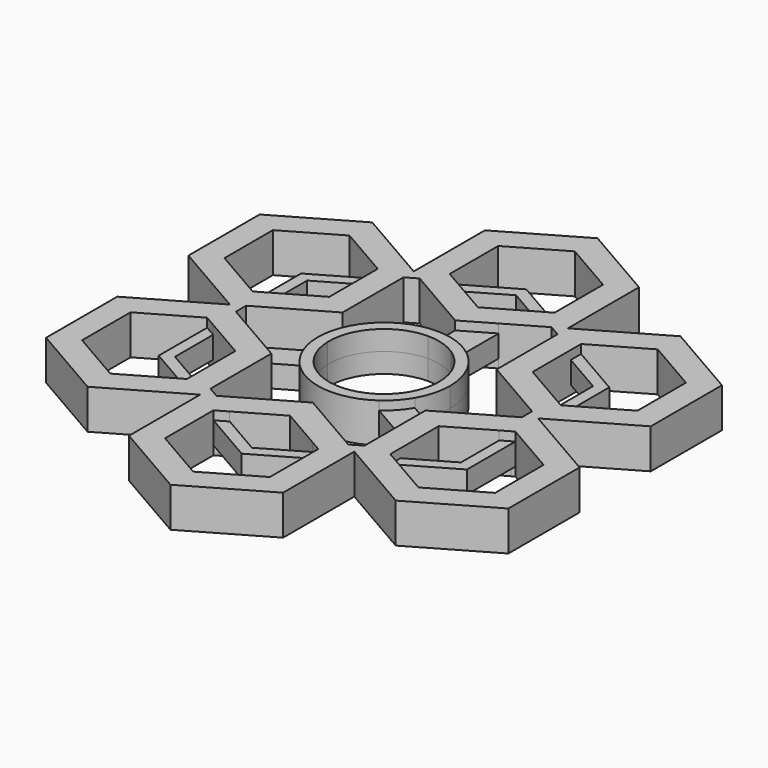
from build123d import *
from build123d import SkipClean  # not in build123d's __all__

# Parameters (mm, degrees)
F1_DEPTH      = 4.572
F1_DEPTH_BACK = 4.572
F4_DEPTH      = 2.032
F6_DEPTH      = 2.032


# Not quite as in the source:
# - after a boolean that leaves OpenCascade's solid faulty, fix() repairs it


with BuildPart() as f1:
    # F0 (on Top) → F1 (new body, two sides)
    with BuildSketch(Plane.XY) as f1_sk:
        Polygon((-23.7368576463, 28.0078895138), (-18.0552325372, 31.2881773), (-35.8352325372, 41.5534650862), (-53.6152325372, 31.2881773), (-53.6152325372, 10.7576017276), (-35.8352325372, 0.4923139414), (-35.8352325372, 7.0528895138), (-47.9336074281, 14.0378895138), (-47.9336074281, 28.0078895138), (-35.8352325372, 34.9928895138), align=None)
        Polygon((-35.8352325372, 7.0528895138), (-35.8352325372, 0.4923139414), (-33.2708004214, 1.9728895138), (-33.2708004214, 8.5334650862), align=None)
        Polygon((-23.7368576463, 25.046738369), (-23.7368576463, 28.0078895138), (-35.8352325372, 21.0228895138), (-35.8352325372, 7.0528895138), (-33.2708004214, 8.5334650862), (-33.2708004214, 19.5423139414), align=None)
        Polygon((-18.0552325372, 28.3270261552), (-18.0552325372, 31.2881773), (-23.7368576463, 28.0078895138), (-23.7368576463, 25.046738369), align=None)
        Polygon((-18.0552325372, 10.7576017276), (-18.0552325372, 28.3270261552), (-23.7368576463, 25.046738369), (-23.7368576463, 14.0378895138), (-33.2708004214, 8.5334650862), (-33.2708004214, 1.9728895138), align=None)
        Polygon((-35.8352325372, 0.4923139414), (-33.2708004214, -0.988261631), (-33.2708004214, 1.9728895138), align=None)
        Polygon((-33.2708004214, -7.5488372033), (-33.2708004214, -0.988261631), (-35.8352325372, 0.4923139414), (-35.8352325372, -6.068261631), align=None)
        Polygon((-35.8352325372, -6.068261631), (-35.8352325372, 0.4923139414), (-53.6152325372, -9.7729738448), (-53.6152325372, -30.3035494172), (-35.8352325372, -40.5688372033), (-18.0552325372, -30.3035494172), (-23.7368576463, -27.023261631), (-35.8352325372, -34.008261631), (-47.9336074281, -27.023261631), (-47.9336074281, -13.053261631), align=None)
        Polygon((-18.0552325372, -9.7729738448), (-24.047449887, -6.3133655448), (-33.2708004214, -0.988261631), (-33.2708004214, -7.5488372033), (-23.7368576463, -13.053261631), (-23.7368576463, -24.0621104862), (-18.0552325372, -27.3423982724), align=None)
        Polygon((-33.2708004214, -18.5576860586), (-33.2708004214, -7.5488372033), (-35.8352325372, -6.068261631), (-35.8352325372, -20.038261631), (-23.7368576463, -27.023261631), (-23.7368576463, -24.0621104862), align=None)
        Polygon((-18.0552325372, -30.3035494172), (-18.0552325372, -27.3423982724), (-23.7368576463, -24.0621104862), (-23.7368576463, -27.023261631), align=None)
        with BuildLine():
            ThreePointArc((-13.4734596909, -7.1276860586), (-14.734134751, -4.324089984), (-15.4065461311, -1.3245374353))
            Line((-15.4065461311, -1.3245374353), (-24.047449887, -6.3133655448))
            Line((-24.047449887, -6.3133655448), (-18.0552325372, -9.7729738448))
            Line((-18.0552325372, -9.7729738448), (-13.4734596909, -7.1276860586))
        make_face()
        with BuildLine():
            ThreePointArc((-11.2737551653, -5.8576860586), (-12.4879200325, -2.9919742416), (-12.9686345677, 0.0829914621))
            Line((-12.9686345677, 0.0829914621), (-15.4065461311, -1.3245374353))
            ThreePointArc((-15.4065461311, -1.3245374353), (-14.734134751, -4.324089984), (-13.4734596909, -7.1276860586))
            Line((-13.4734596909, -7.1276860586), (-11.2737551653, -5.8576860586))
        make_face()
        with BuildLine():
            ThreePointArc((-12.9686345677, 0.0829914621), (-9.3990583654, 9.3266674693), (-0.2752325372, 13.1923139414))
            Line((-0.2752325372, 13.1923139414), (-0.2752325372, 15.7323139414))
            ThreePointArc((-0.2752325372, 15.7323139414), (-11.6758117984, 10.6058886067), (-15.4065461311, -1.3245374353))
            Line((-15.4065461311, -1.3245374353), (-12.9686345677, 0.0829914621))
        make_face()
        with BuildLine():
            ThreePointArc((-0.2752325372, 13.1923139414), (3.3044248707, 12.677388945), (6.5938058883, 11.1743695071))
            Line((6.5938058883, 11.1743695071), (6.5938058883, 14.0965012052))
            ThreePointArc((6.5938058883, 14.0965012052), (3.2553330053, 15.3177214215), (-0.2752325372, 15.7323139414))
            Line((-0.2752325372, 15.7323139414), (-0.2752325372, 13.1923139414))
        make_face()
        with BuildLine():
            ThreePointArc((-0.2752325372, 15.7323139414), (3.2553330053, 15.3177214215), (6.5938058883, 14.0965012052))
            Line((6.5938058883, 14.0965012052), (6.5938058883, 24.9887306979))
            Line((6.5938058883, 24.9887306979), (-0.2752325372, 21.0228895138))
            Line((-0.2752325372, 21.0228895138), (-0.2752325372, 15.7323139414))
        make_face()
        with BuildLine():
            ThreePointArc((6.5938058883, 11.1743695071), (10.8721166545, 6.5772630782), (12.4247674628, 0.4923139414))
            ThreePointArc((12.4247674628, 0.4923139414), (11.9920254567, -2.7946879314), (10.7232900908, -5.8576860586))
            Line((10.7232900908, -5.8576860586), (12.9229946165, -7.1276860586))
            ThreePointArc((12.9229946165, -7.1276860586), (14.4454770554, -3.4520883059), (14.9647674628, 0.4923139414))
            ThreePointArc((14.9647674628, 0.4923139414), (12.7044004623, 8.4789732679), (6.5938058883, 14.0965012052))
            Line((6.5938058883, 14.0965012052), (6.5938058883, 11.1743695071))
        make_face()
        with BuildLine():
            Line((12.9229946165, -7.1276860586), (10.7232900908, -5.8576860586))
            ThreePointArc((10.7232900908, -5.8576860586), (8.6919237144, -8.5010229676), (6.0426758858, -10.5246744474))
            Line((6.0426758858, -10.5246744474), (8.5189644271, -11.9543603033))
            ThreePointArc((8.5189644271, -11.9543603033), (10.9826924808, -9.779819444), (12.9229946165, -7.1276860586))
        make_face()
        with BuildLine():
            Line((8.5189644271, -11.9543603033), (6.0426758858, -10.5246744474))
            ThreePointArc((6.0426758858, -10.5246744474), (-3.5801126393, -11.7701396267), (-11.2737551653, -5.8576860586))
            Line((-11.2737551653, -5.8576860586), (-13.4734596909, -7.1276860586))
            ThreePointArc((-13.4734596909, -7.1276860586), (-3.542198491, -14.3934018108), (8.5189644271, -11.9543603033))
        make_face()
        with BuildLine():
            Line((17.5047674628, -9.7729738448), (12.9229946165, -7.1276860586))
            ThreePointArc((12.9229946165, -7.1276860586), (10.9826924808, -9.779819444), (8.5189644271, -11.9543603033))
            Line((8.5189644271, -11.9543603033), (17.5047674628, -17.1423161048))
            Line((17.5047674628, -17.1423161048), (17.5047674628, -9.7729738448))
        make_face()
        Polygon((-15.4908004214, -28.8229738448), (-18.0552325372, -27.3423982724), (-18.0552325372, -30.3035494172), align=None)
        Polygon((-15.4908004214, -28.8229738448), (-18.0552325372, -30.3035494172), (-12.3736074281, -33.5838372033), (-9.8091753123, -32.103261631), align=None)
        Polygon((9.2587102378, -32.103261631), (14.940335347, -28.8229738448), (-0.2752325372, -20.038261631), (-15.4908004214, -28.8229738448), (-9.8091753123, -32.103261631), (-0.2752325372, -26.5988372033), align=None)
        Polygon((17.5047674628, -50.8341249895), (17.5047674628, -30.3035494172), (11.8231423537, -33.5838372033), (11.8231423537, -47.5538372033), (-0.2752325372, -54.5388372033), (-12.3736074281, -47.5538372033), (-12.3736074281, -33.5838372033), (-18.0552325372, -30.3035494172), (-18.0552325372, -50.8341249895), (-0.2752325372, -61.0994127757), align=None)
        Polygon((-0.2752325372, -40.5688372033), (11.8231423537, -33.5838372033), (9.2587102378, -32.103261631), (-0.2752325372, -37.6076860586), (-9.8091753123, -32.103261631), (-12.3736074281, -33.5838372033), align=None)
        Polygon((11.8231423537, -33.5838372033), (17.5047674628, -30.3035494172), (14.940335347, -28.8229738448), (9.2587102378, -32.103261631), align=None)
        Polygon((32.720335347, -0.988261631), (17.5047674628, -9.7729738448), (17.5047674628, -17.1423161048), (17.5047674628, -27.3423982724), (23.1863925719, -24.0621104862), (23.1863925719, -13.053261631), (32.720335347, -7.5488372033), align=None)
        Polygon((23.1863925719, -24.0621104862), (17.5047674628, -27.3423982724), (17.5047674628, -30.3035494172), (23.1863925719, -27.023261631), align=None)
        Polygon((17.5047674628, -30.3035494172), (17.5047674628, -27.3423982724), (14.940335347, -28.8229738448), align=None)
        Polygon((35.2847674628, 0.4923139414), (32.720335347, -0.988261631), (32.720335347, -7.5488372033), (35.2847674628, -6.068261631), align=None)
        Polygon((53.0647674628, -9.7729738448), (35.2847674628, 0.4923139414), (35.2847674628, -6.068261631), (47.3831423537, -13.053261631), (47.3831423537, -27.023261631), (35.2847674628, -34.008261631), (23.1863925719, -27.023261631), (17.5047674628, -30.3035494172), (35.2847674628, -40.5688372033), (53.0647674628, -30.3035494172), align=None)
        Polygon((35.2847674628, -6.068261631), (32.720335347, -7.5488372033), (32.720335347, -18.5576860586), (23.1863925719, -24.0621104862), (23.1863925719, -27.023261631), (35.2847674628, -20.038261631), align=None)
        Polygon((32.720335347, 1.9728895138), (32.720335347, -0.988261631), (35.2847674628, 0.4923139414), align=None)
        Polygon((32.720335347, 1.9728895138), (35.2847674628, 0.4923139414), (35.2847674628, 7.0528895138), (32.720335347, 8.5334650862), align=None)
        Polygon((23.1863925719, 25.046738369), (17.5047674628, 28.3270261552), (17.5047674628, 10.7576017276), (32.720335347, 1.9728895138), (32.720335347, 8.5334650862), (23.1863925719, 14.0378895138), align=None)
        Polygon((35.2847674628, 41.5534650862), (17.5047674628, 31.2881773), (23.1863925719, 28.0078895138), (35.2847674628, 34.9928895138), (47.3831423537, 28.0078895138), (47.3831423537, 14.0378895138), (35.2847674628, 7.0528895138), (35.2847674628, 0.4923139414), (53.0647674628, 10.7576017276), (53.0647674628, 31.2881773), align=None)
        Polygon((35.2847674628, 21.0228895138), (23.1863925719, 28.0078895138), (23.1863925719, 25.046738369), (32.720335347, 19.5423139414), (32.720335347, 8.5334650862), (35.2847674628, 7.0528895138), align=None)
        Polygon((23.1863925719, 28.0078895138), (17.5047674628, 31.2881773), (17.5047674628, 28.3270261552), (23.1863925719, 25.046738369), align=None)
        Polygon((17.5047674628, 31.2881773), (14.940335347, 29.8076017276), (17.5047674628, 28.3270261552), align=None)
        Polygon((9.2587102378, 33.0878895138), (14.940335347, 29.8076017276), (17.5047674628, 31.2881773), (11.8231423537, 34.5684650862), align=None)
        Polygon((-0.2752325372, 21.0228895138), (6.5938058883, 24.9887306979), (14.940335347, 29.8076017276), (9.2587102378, 33.0878895138), (-0.2752325372, 27.5834650862), (-9.8091753123, 33.0878895138), (-15.4908004214, 29.8076017276), align=None)
        Polygon((11.8231423537, 34.5684650862), (17.5047674628, 31.2881773), (17.5047674628, 51.8187528724), (-0.2752325372, 62.0840406586), (-18.0552325372, 51.8187528724), (-18.0552325372, 31.2881773), (-12.3736074281, 34.5684650862), (-12.3736074281, 48.5384650862), (-0.2752325372, 55.5234650862), (11.8231423537, 48.5384650862), align=None)
        Polygon((-0.2752325372, 38.5923139414), (9.2587102378, 33.0878895138), (11.8231423537, 34.5684650862), (-0.2752325372, 41.5534650862), (-12.3736074281, 34.5684650862), (-9.8091753123, 33.0878895138), align=None)
        Polygon((-18.0552325372, 31.2881773), (-15.4908004214, 29.8076017276), (-9.8091753123, 33.0878895138), (-12.3736074281, 34.5684650862), align=None)
        Polygon((-18.0552325372, 28.3270261552), (-15.4908004214, 29.8076017276), (-18.0552325372, 31.2881773), align=None)
    extrude(amount=F1_DEPTH)
    extrude(f1_sk.sketch, amount=-F1_DEPTH_BACK)

    # F3 (on face) → F4 (cut)
    with BuildSketch(Plane.XY.offset(4.572)):
        Polygon((-33.2708004214, 19.5423139414), (-23.7368576463, 25.046738369), (-23.7368576463, 28.0078895138), (-35.8352325372, 21.0228895138), (-35.8352325372, 7.0528895138), (-33.2708004214, 8.5334650862), align=None)
        Polygon((-0.2752325372, 38.5923139414), (9.2587102378, 33.0878895138), (11.8231423537, 34.5684650862), (-0.2752325372, 41.5534650862), (-12.3736074281, 34.5684650862), (-9.8091753123, 33.0878895138), align=None)
        Polygon((35.2847674628, 21.0228895138), (23.1863925719, 28.0078895138), (23.1863925719, 25.046738369), (32.720335347, 19.5423139414), (32.720335347, 8.5334650862), (35.2847674628, 7.0528895138), align=None)
        Polygon((35.2847674628, -6.068261631), (32.720335347, -7.5488372033), (32.720335347, -18.5576860586), (23.1863925719, -24.0621104862), (23.1863925719, -27.023261631), (35.2847674628, -20.038261631), align=None)
        Polygon((-0.2752325372, -40.5688372033), (11.8231423537, -33.5838372033), (9.2587102378, -32.103261631), (-0.2752325372, -37.6076860586), (-9.8091753123, -32.103261631), (-12.3736074281, -33.5838372033), align=None)
        Polygon((-33.2708004214, -18.5576860586), (-33.2708004214, -7.5488372033), (-35.8352325372, -6.068261631), (-35.8352325372, -20.038261631), (-23.7368576463, -27.023261631), (-23.7368576463, -24.0621104862), align=None)
        with BuildLine():
            Line((17.5047674628, -9.7729738448), (12.9229946165, -7.1276860586))
            ThreePointArc((12.9229946165, -7.1276860586), (10.9826924808, -9.779819444), (8.5189644271, -11.9543603033))
            Line((8.5189644271, -11.9543603033), (17.5047674628, -17.1423161048))
            Line((17.5047674628, -17.1423161048), (17.5047674628, -9.7729738448))
        make_face()
        with BuildLine():
            ThreePointArc((-13.4734596909, -7.1276860586), (-14.734134751, -4.324089984), (-15.4065461311, -1.3245374353))
            Line((-15.4065461311, -1.3245374353), (-24.047449887, -6.3133655448))
            Line((-24.047449887, -6.3133655448), (-18.0552325372, -9.7729738448))
            Line((-18.0552325372, -9.7729738448), (-13.4734596909, -7.1276860586))
        make_face()
        with BuildLine():
            ThreePointArc((-0.2752325372, 15.7323139414), (3.2553330053, 15.3177214215), (6.5938058883, 14.0965012052))
            Line((6.5938058883, 14.0965012052), (6.5938058883, 24.9887306979))
            Line((6.5938058883, 24.9887306979), (-0.2752325372, 21.0228895138))
            Line((-0.2752325372, 21.0228895138), (-0.2752325372, 15.7323139414))
        make_face()
    with SkipClean():  # cleaning this boolean's faces spoils the solid; the shape is the same uncleaned
        extrude(amount=-F4_DEPTH, mode=Mode.SUBTRACT)

    # F2 (on face) → F6 (cut)
    with BuildSketch(Plane(origin=(0, 0, -4.572), x_dir=(1, 0, 0), z_dir=(0, 0, -1))):
        Polygon((-23.7368576463, 26.2296947263), (-23.7368576463, 27.023261631), (-29.9010039346, 23.4643901121), (-35.8352325372, 20.038261631), (-35.8352325372, 13.1860046687), (-35.8352325372, 6.068261631), (-35.1479834382, 6.4650450833), (-33.2708004214, 7.5488372033), (-33.2708004214, 12.7668753249), (-33.2708004214, 18.5576860586), (-28.2558112175, 21.4530914254), (-23.7368576463, 24.0621104862), align=None)
        Polygon((-35.1479834382, -7.4496729661), (-35.8352325372, -7.0528895138), (-35.8352325372, -14.1706325515), (-35.8352325372, -21.0228895138), (-23.7368576463, -28.0078895138), (-23.7368576463, -27.2143226092), (-23.7368576463, -25.046738369), (-28.2558112175, -22.4377193083), (-33.2708004214, -19.5423139414), (-33.2708004214, -13.7515032077), (-33.2708004214, -8.5334650862), align=None)
        Polygon((-11.6863583291, -34.1716816339), (-12.3736074281, -34.5684650862), (-6.2094611398, -38.1273366051), (-0.2752325372, -41.5534650862), (11.8231423537, -34.5684650862), (11.1358932546, -34.1716816339), (9.2587102378, -33.0878895138), (4.7397566667, -35.6969085746), (-0.2752325372, -38.5923139414), (-5.2902217411, -35.6969085746), (-9.8091753123, -33.0878895138), align=None)
        Polygon((35.2847674628, -21.0228895138), (35.2847674628, -7.0528895138), (34.5975183638, -7.4496729661), (32.720335347, -8.5334650862), (32.720335347, -13.7515032077), (32.720335347, -19.5423139414), (27.7053461431, -22.4377193083), (23.1863925719, -25.046738369), (23.1863925719, -27.2143226092), (23.1863925719, -28.0078895138), (29.3505388602, -24.4490179949), align=None)
        Polygon((35.2847674628, 20.038261631), (23.1863925719, 27.023261631), (23.1863925719, 26.2296947263), (23.1863925719, 24.0621104862), (27.7053461431, 21.4530914254), (32.720335347, 18.5576860586), (32.720335347, 12.7668753249), (32.720335347, 7.5488372033), (34.5975183638, 6.4650450833), (35.2847674628, 6.068261631), (35.2847674628, 13.1860046687), align=None)
        Polygon((-10.7527325372, 34.5196497579), (-12.3736074281, 33.5838372033), (-11.6863583291, 33.187053751), (-9.8091753123, 32.103261631), (-9.2324389334, 32.4362405346), (-5.2902217411, 34.7122806917), (-0.2752325372, 37.6076860586), (4.7397566667, 34.7122806917), (8.6819738589, 32.4362405346), (9.2587102378, 32.103261631), (11.1358932546, 33.187053751), (11.8231423537, 33.5838372033), (10.2022674628, 34.5196497579), (5.6589960654, 37.1427087222), (-0.2752325372, 40.5688372033), (-6.2094611398, 37.1427087222), align=None)
        with BuildLine():
            Line((-13.4734596909, 7.1276860586), (-18.0552325372, 9.7729738448))
            Line((-18.0552325372, 9.7729738448), (-24.047449887, 6.3133655448))
            Line((-24.047449887, 6.3133655448), (-21.8255069655, 5.0305262009))
            Line((-21.8255069655, 5.0305262009), (-15.4065461311, 1.3245374353))
            ThreePointArc((-15.4065461311, 1.3245374353), (-14.734134751, 4.324089984), (-13.4734596909, 7.1276860586))
        make_face()
        with BuildLine():
            Line((15.1946185934, 15.8085510332), (8.5189644271, 11.9543603033))
            ThreePointArc((8.5189644271, 11.9543603033), (10.9826924808, 9.779819444), (12.9229946165, 7.1276860586))
            Line((12.9229946165, 7.1276860586), (17.5047674628, 9.7729738448))
            Line((17.5047674628, 9.7729738448), (17.5047674628, 17.1423161048))
            Line((17.5047674628, 17.1423161048), (15.1946185934, 15.8085510332))
        make_face()
        with BuildLine():
            ThreePointArc((6.5938058883, -14.0965012052), (3.2553330053, -15.3177214215), (-0.2752325372, -15.7323139414))
            Line((-0.2752325372, -15.7323139414), (-0.2752325372, -21.0228895138))
            Line((-0.2752325372, -21.0228895138), (6.5938058883, -24.9887306979))
            Line((6.5938058883, -24.9887306979), (6.5938058883, -22.2060920231))
            Line((6.5938058883, -22.2060920231), (6.5938058883, -14.0965012052))
        make_face()
    extrude(amount=-F6_DEPTH, mode=Mode.SUBTRACT)

    add(f1.part.fix(), mode=Mode.REPLACE)


solid = f1.part
